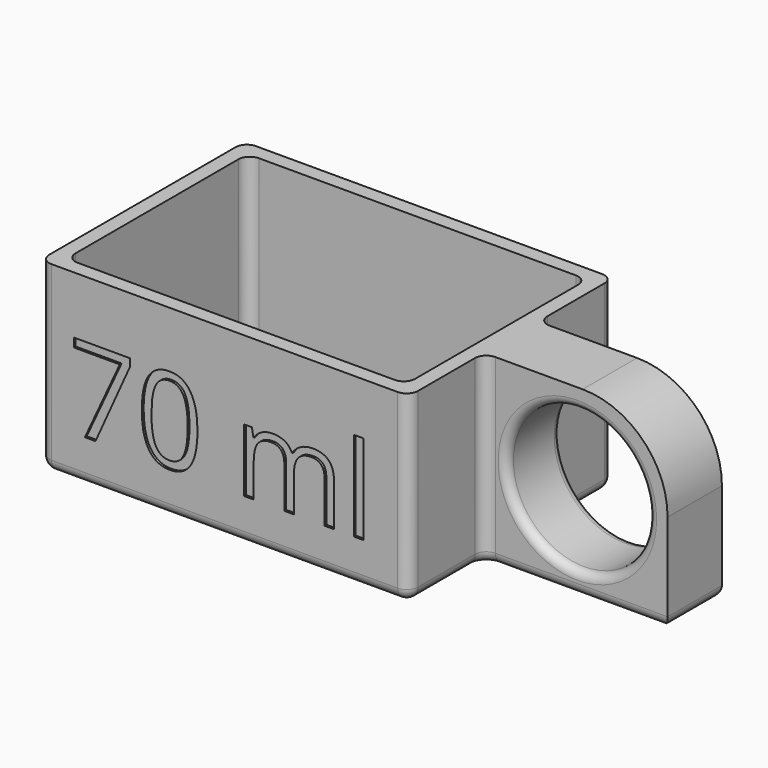
from build123d import *

# Parameters (mm, degrees)
F0_W         = 65.14
F0_H         = 45.14
F0_W_2       = 60
F0_H_2       = 40
F1_DEPTH     = 30
F2_DEPTH     = 2.5
F3_R         = 2
F4_R         = 12.5
F5_DEPTH     = 6
F6_T1_DEPTH  = 32.5
F6_T3_DEPTH  = 12.57
F6_T5_DEPTH  = 35.43
F6_T7_DEPTH  = 22
F6_T9_DEPTH  = 12.57
F6_S13_W     = 2.04
F6_S13_H     = 2.04
F6_T14_DEPTH = 2.04
F6_S19_W     = 2.04
F6_S19_H     = 2.04
F6_T20_DEPTH = 2.04
F6_T24_ANGLE = 90
F6_T26_ANGLE = 90
F7_TEXT_SIZE = 20.8333333333
F8_DEPTH     = 0.4
F9_TEXT_SIZE = 20.8333333333
F10_DEPTH    = 0.4
F11_R        = 1.5


# Not quite as in the source:
# - a fillet or chamfer that OpenCascade refuses, or shapes differently, is made with other operations: its cross-section is extruded or revolved along the edge and cut away or added
# - Text() gives the source's letters only with a copy of the font that has no kerning and outlines rounded to 1/6400 em; it was checked with that copy


with BuildPart() as f1:
    # F0 (on Top) → F1 (new body)
    with BuildSketch(Plane.XY):
        Rectangle(F0_W, F0_H)
        Rectangle(F0_W_2, F0_H_2, mode=Mode.SUBTRACT)
    extrude(amount=F1_DEPTH)

    # F0 (on Top) → F2 (join)
    with BuildSketch(Plane.XY):
        Rectangle(F0_W, F0_H)
        Rectangle(F0_W_2, F0_H_2, mode=Mode.SUBTRACT)
        Rectangle(F0_W_2, F0_H_2)
    extrude(amount=-F2_DEPTH)

    # F3
    f3_edges = [f1.edges().sort_by_distance(p)[0] for p in [
        (-30, 20, 15),
        (-30, 0, 0),
        (0, 20, 0),
        (-30, -20, 15),
        (30, 20, 15),
        (30, 0, 0),
        (0, -20, 0),
        (30, -20, 15),
        (32.57, -22.57, 13.75),
        (32.57, 22.57, 13.75),
        (-32.57, -22.57, 13.75),
        (-32.57, 22.57, 13.75),
        (0, -22.57, -2.5),
        (-32.57, 0, -2.5),
        (0, 22.57, -2.5),
    ]]
    fillet(f3_edges, radius=F3_R)

    # F4 (on Front) → F5 (join, symmetric)
    with BuildSketch(Plane.XZ):
        with BuildLine():
            Line((50, 30), (32.57, 30))
            Line((32.57, 30), (32.57, -2.5))
            Line((32.57, -2.5), (65, -2.5))
            Line((65, -2.5), (65, 15))
            ThreePointArc((65, 15), (60.6066017178, 25.6066017178), (50, 30))
        make_face()
        with Locations((49.07, 14)):
            Circle(F4_R, mode=Mode.SUBTRACT)
    extrude(amount=F5_DEPTH, both=True)

    # F6: fillet of radius 2 on 7 edges, made by hand

    # F6_s2 → F6_t1 (join)
    with BuildSketch(Plane.XY.offset(-2.5)):
        with BuildLine():
            ThreePointArc((32.57, -8), (33.1557864376, -6.5857864376), (34.57, -6))
            Line((34.57, -6), (32.57, -6))
            Line((32.57, -6), (32.57, -8))
        make_face()
        with BuildLine():
            ThreePointArc((32.57, 8), (33.1557864376, 6.5857864376), (34.57, 6))
            Line((34.57, 6), (32.57, 6))
            Line((32.57, 6), (32.57, 8))
        make_face()
    extrude(amount=F6_T1_DEPTH)

    # F6_s4 → F6_t3 (cut)
    with BuildSketch(Plane.XZ.offset(-20.57)):
        with BuildLine():
            ThreePointArc((32.57, -0.5), (31.9842135624, -1.9142135624), (30.57, -2.5))
            Line((30.57, -2.5), (32.57, -2.5))
            Line((32.57, -2.5), (32.57, -0.5))
        make_face()
    extrude(amount=F6_T3_DEPTH, mode=Mode.SUBTRACT)

    # F6_s6 → F6_t5 (cut)
    with BuildSketch(Plane.YZ.offset(34.57)):
        with BuildLine():
            ThreePointArc((6, -0.5), (5.4142135624, -1.9142135624), (4, -2.5))
            Line((4, -2.5), (6, -2.5))
            Line((6, -2.5), (6, -0.5))
        make_face()
        with BuildLine():
            ThreePointArc((-6, -0.5), (-5.4142135624, -1.9142135624), (-4, -2.5))
            Line((-4, -2.5), (-6, -2.5))
            Line((-6, -2.5), (-6, -0.5))
        make_face()
    extrude(amount=F6_T5_DEPTH, mode=Mode.SUBTRACT)

    # F6_s8 → F6_t7 (cut)
    with BuildSketch(Plane.XZ.offset(-11)):
        with BuildLine():
            ThreePointArc((63, -2.5), (64.4142135624, -1.9142135624), (65, -0.5))
            Line((65, -0.5), (65, -2.5))
            Line((65, -2.5), (63, -2.5))
        make_face()
    extrude(amount=F6_T7_DEPTH, mode=Mode.SUBTRACT)

    # F6_s10 → F6_t9 (cut)
    with BuildSketch(Plane.XZ.offset(8)):
        with BuildLine():
            ThreePointArc((32.57, -0.5), (31.9842135624, -1.9142135624), (30.57, -2.5))
            Line((30.57, -2.5), (32.57, -2.5))
            Line((32.57, -2.5), (32.57, -0.5))
        make_face()
    extrude(amount=F6_T9_DEPTH, mode=Mode.SUBTRACT)


with BuildPart() as f6_tool12:
    # F6_s13 → F6_t14 (new body)
    with BuildSketch(Plane.YZ.offset(30.57)):
        with Locations((-21.59, -1.52)):
            Rectangle(F6_S13_W, F6_S13_H)
    extrude(amount=F6_T14_DEPTH)

    # F6_s15 → F6_t16 (revolve, cut)
    with BuildSketch(Plane(origin=(30.57, -20.57, -0.5), x_dir=(0, 0.7071067812, 0.7071067812), z_dir=(0, 0.7071067812, -0.7071067812))):
        with BuildLine():
            ThreePointArc((0, -2), (2, 0), (0, 2))
            Line((0, 2), (0, -2))
        make_face()
    revolve(axis=Axis((30.57, -20.57, -0.5), (1, 0, 0)), mode=Mode.SUBTRACT)


with BuildPart() as f1_1:
    add(f1.part)

    # F6_t11: cut F6_tool12
    add(f6_tool12.part, mode=Mode.SUBTRACT)


with BuildPart() as f6_tool18:
    # F6_s19 → F6_t20 (new body)
    with BuildSketch(Plane.YZ.offset(30.57)):
        with Locations((21.59, -1.52)):
            Rectangle(F6_S19_W, F6_S19_H)
    extrude(amount=F6_T20_DEPTH)

    # F6_s21 → F6_t22 (revolve, cut)
    with BuildSketch(Plane(origin=(30.57, 20.57, -0.5), x_dir=(0, -0.7071067812, 0.7071067812), z_dir=(0, 0.7071067812, 0.7071067812))):
        with BuildLine():
            ThreePointArc((0, -2), (2, 0), (0, 2))
            Line((0, 2), (0, -2))
        make_face()
    revolve(axis=Axis((30.57, 20.57, -0.5), (1, 0, 0)), mode=Mode.SUBTRACT)


with BuildPart() as f1_2:
    add(f1_1.part)

    # F6_t17: cut F6_tool18
    add(f6_tool18.part, mode=Mode.SUBTRACT)

    # F6_s23 → F6_t24 (revolve, cut)
    with BuildSketch(Plane.XZ.offset(8)):
        with BuildLine():
            ThreePointArc((30.57, -2.5), (31.9842135624, -1.9142135624), (32.57, -0.5))
            Line((32.57, -0.5), (32.57, -2.5))
            Line((32.57, -2.5), (30.57, -2.5))
        make_face()
    revolve(axis=Axis((34.57, -8, -2.5), (0, 0, -1)), revolution_arc=F6_T24_ANGLE, mode=Mode.SUBTRACT)

    # F6_s25 → F6_t26 (revolve, cut)
    with BuildSketch(Plane.XZ.offset(-8)):
        with BuildLine():
            ThreePointArc((30.57, -2.5), (31.9842135624, -1.9142135624), (32.57, -0.5))
            Line((32.57, -0.5), (32.57, -2.5))
            Line((32.57, -2.5), (30.57, -2.5))
        make_face()
    revolve(axis=Axis((34.57, 8, -2.5), (0, 0, 1)), revolution_arc=F6_T26_ANGLE, mode=Mode.SUBTRACT)

    # F7 (on face) → F8 (cut)
    with BuildSketch(Plane(origin=(0, 22.57, 0), x_dir=(-1, 0, 0), z_dir=(0, 1, 0))):
        with Locations((-27.57, 5)):
            Text('70 ml', F7_TEXT_SIZE, font='Open Sans', text_align=(TextAlign.LEFT, TextAlign.BOTTOM))
    extrude(amount=-F8_DEPTH, mode=Mode.SUBTRACT)

    # F9 (on face) → F10 (cut)
    with BuildSketch(Plane.XZ.offset(22.57)):
        with Locations((-27.57, 5)):
            Text('70 ml', F9_TEXT_SIZE, font='Open Sans', text_align=(TextAlign.LEFT, TextAlign.BOTTOM))
    extrude(amount=-F10_DEPTH, mode=Mode.SUBTRACT)

    # F11
    f11_edges = [f1_2.edges().sort_by_distance(p)[0] for p in [
        (36.57, -6, 14),
        (61.57, 0, 14),
        (36.57, 6, 14),
    ]]
    fillet(f11_edges, radius=F11_R)


solid = f1_2.part
